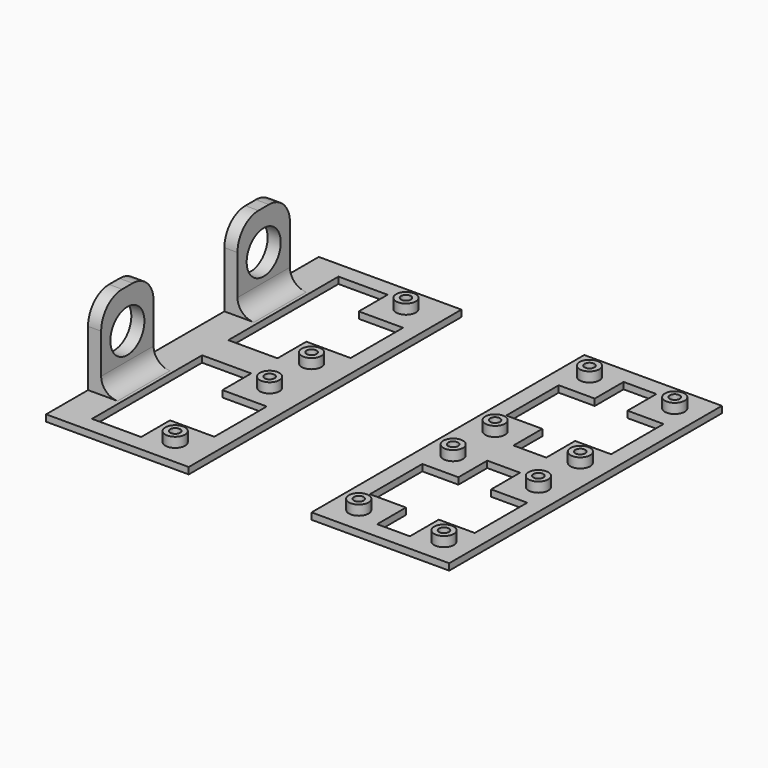
from build123d import *

# Parameters (mm, degrees)
F0_R     = 3
F0_R_2   = 1.5
F1_DEPTH = 2
F0_W     = 43.5258374241
F0_H     = 104
F2_DEPTH = 5
F4_R     = 6.5
F5_DEPTH = 4
F6_R     = 5
F7_R     = 8


# Not quite as in the source:
# - a feature names something its author has since deleted; it is built from what else it names


with BuildPart() as f1:
    # F0 (on Top) → F1 (new body)
    with BuildSketch(Plane.XY):
        Polygon((21, 52), (20, 52), (-20, 52), (-21, 52), (-21, -52), (-20, -52), (20, -52), (21, -52), align=None)
        with Locations((-13, -44)):
            Circle(F0_R, mode=Mode.SUBTRACT)
        with Locations((13, -44)):
            Circle(F0_R, mode=Mode.SUBTRACT)
        with Locations((-13, -8)):
            Circle(F0_R, mode=Mode.SUBTRACT)
        Polygon((-5, -16), (-5, -5), (5, -5), (5, -16), (16, -16), (16, -36), (5, -36), (5, -47), (-5, -47), (-5, -36), (-16, -36), (-16, -16), align=None, mode=Mode.SUBTRACT)
        with Locations((13, -8)):
            Circle(F0_R, mode=Mode.SUBTRACT)
        with Locations((-13, 8)):
            Circle(F0_R, mode=Mode.SUBTRACT)
        with Locations((13, 8)):
            Circle(F0_R, mode=Mode.SUBTRACT)
        with Locations((-13, 44)):
            Circle(F0_R, mode=Mode.SUBTRACT)
        Polygon((-5, 36), (-5, 47), (5, 47), (5, 36), (16, 36), (16, 16), (5, 16), (5, 5), (-5, 5), (-5, 16), (-16, 16), (-16, 36), align=None, mode=Mode.SUBTRACT)
        with Locations((13, 44)):
            Circle(F0_R, mode=Mode.SUBTRACT)
        with Locations((-13, 8)):
            Circle(F0_R)
        with Locations((-13, 8)):
            Circle(F0_R_2, mode=Mode.SUBTRACT)
        with Locations((-13, 44)):
            Circle(F0_R)
        with Locations((-13, 44)):
            Circle(F0_R_2, mode=Mode.SUBTRACT)
    extrude(amount=F1_DEPTH)

    # F0 (on Top) → F2, piece 2 (join)
    with BuildSketch(Plane.XY):
        with Locations((-13, 8)):
            Circle(F0_R)
        with Locations((-13, 8)):
            Circle(F0_R_2, mode=Mode.SUBTRACT)
        with Locations((-13, 44)):
            Circle(F0_R)
        with Locations((-13, 44)):
            Circle(F0_R_2, mode=Mode.SUBTRACT)
        with Locations((13, 44)):
            Circle(F0_R)
        with Locations((13, 44)):
            Circle(F0_R_2, mode=Mode.SUBTRACT)
        with Locations((13, 8)):
            Circle(F0_R)
        with Locations((13, 8)):
            Circle(F0_R_2, mode=Mode.SUBTRACT)
        with Locations((-13, -8)):
            Circle(F0_R)
        with Locations((-13, -8)):
            Circle(F0_R_2, mode=Mode.SUBTRACT)
        with Locations((13, -8)):
            Circle(F0_R)
        with Locations((13, -8)):
            Circle(F0_R_2, mode=Mode.SUBTRACT)
        with Locations((-13, -44)):
            Circle(F0_R)
        with Locations((-13, -44)):
            Circle(F0_R_2, mode=Mode.SUBTRACT)
        with Locations((13, -44)):
            Circle(F0_R)
        with Locations((13, -44)):
            Circle(F0_R_2, mode=Mode.SUBTRACT)
    extrude(amount=F2_DEPTH)


with BuildPart() as f1b:
    # F0 (on Top) → F1, piece 2 (new body)
    with BuildSketch(Plane.XY):
        with Locations((-80.2370812879, 0)):
            Rectangle(F0_W, F0_H)
        with Locations((-69, -44)):
            Circle(F0_R, mode=Mode.SUBTRACT)
        Polygon((-77, -47), (-92, -47), (-92, -5), (-77, -5), (-77, -16), (-63.4741625759, -16), (-63.4741625759, -36), (-77, -36), align=None, mode=Mode.SUBTRACT)
        with Locations((-69, -8)):
            Circle(F0_R, mode=Mode.SUBTRACT)
        with Locations((-69, 8)):
            Circle(F0_R, mode=Mode.SUBTRACT)
        Polygon((-92, 47), (-77, 47), (-77, 36), (-63.4741625759, 36), (-63.4741625759, 16), (-77, 16), (-77, 5), (-92, 5), align=None, mode=Mode.SUBTRACT)
        with Locations((-69, 44)):
            Circle(F0_R, mode=Mode.SUBTRACT)
    extrude(amount=F1_DEPTH)

    # F0 (on Top) → F2 (join)
    with BuildSketch(Plane.XY):
        with Locations((-69, 44)):
            Circle(F0_R)
        with Locations((-69, 44)):
            Circle(F0_R_2, mode=Mode.SUBTRACT)
        with Locations((-69, 8)):
            Circle(F0_R)
        with Locations((-69, 8)):
            Circle(F0_R_2, mode=Mode.SUBTRACT)
        with Locations((-69, -8)):
            Circle(F0_R)
        with Locations((-69, -8)):
            Circle(F0_R_2, mode=Mode.SUBTRACT)
        with Locations((-69, -44)):
            Circle(F0_R)
        with Locations((-69, -44)):
            Circle(F0_R_2, mode=Mode.SUBTRACT)
    extrude(amount=F2_DEPTH)

    # F4 (on face) → F5 (join)
    with BuildSketch(Plane(origin=(-102, 0, 0), x_dir=(0, -1, 0), z_dir=(-1, 0, 0))):
        Polygon((-16, 27.1253478074), (-35.9944990628, 27.1253478074), (-35.9944990628, 0), (-16, 0.4690492824), align=None)
        with Locations((-25.9972495314, 15.1253478074)):
            Circle(F4_R, mode=Mode.SUBTRACT)
        Polygon((16, 0.4690492824), (35.9944990628, 0), (35.9944990628, 27.1253478074), (16, 27.1253478074), align=None)
        with Locations((25.9972495314, 15.1253478074)):
            Circle(F4_R, mode=Mode.SUBTRACT)
    extrude(amount=-F5_DEPTH)

    # F6
    f6_edges = [f1b.edges().sort_by_distance(p)[0] for p in [
        (-98, 25.99725, 2),
        (-98, -25.99725, 2),
    ]]
    fillet(f6_edges, radius=F6_R)

    # F7
    f7_edges = [f1b.edges().sort_by_distance(p)[0] for p in [
        (-100, 35.994499, 27.125348),
        (-100, -16, 27.125348),
        (-100, 16, 27.125348),
        (-100, -35.994499, 27.125348),
    ]]
    fillet(f7_edges, radius=F7_R)


solid = Compound([f1.part, f1b.part])
